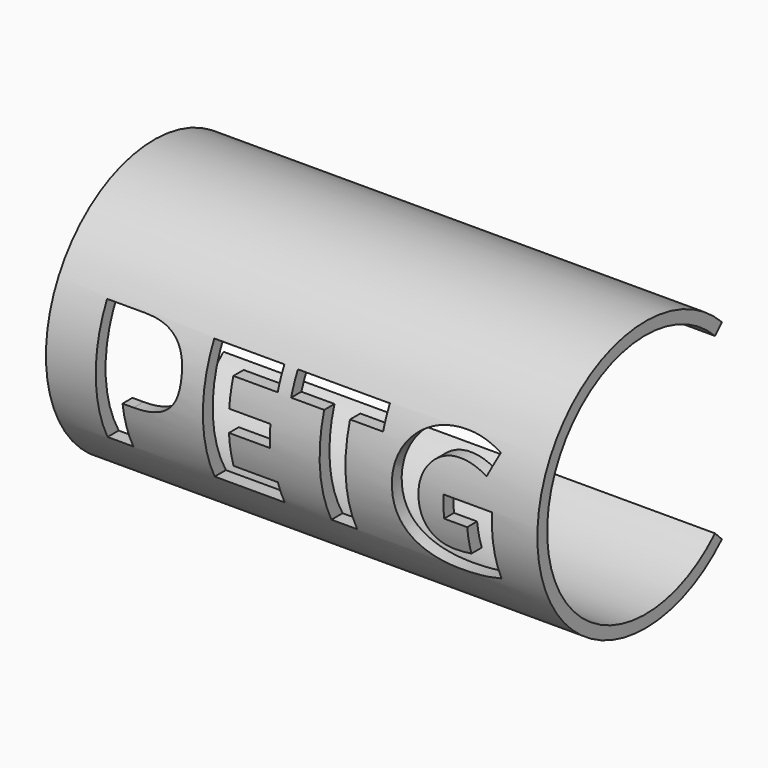
from build123d import *

# Parameters (mm, degrees)
F1_DEPTH     = 50.8
F3_TEXT_SIZE = 17.6388888889
F4_DEPTH     = 35.2792817332


# Not quite as in the source:
# - Text() gives the source's letters only with a copy of the font that has no kerning and outlines rounded to 1/6400 em; it was checked with that copy


with BuildPart() as f1:
    # F0 (on Right) → F1 (new body)
    with BuildSketch(Plane.YZ):
        with BuildLine():
            ThreePointArc((8.9802561211, -8.9802561211), (-12.7, 0), (8.9802561211, 8.9802561211))
            Line((8.9802561211, 8.9802561211), (9.8782817332, 9.8782817332))
            ThreePointArc((9.8782817332, 9.8782817332), (-13.97, 0), (9.8782817332, -9.8782817332))
            Line((9.8782817332, -9.8782817332), (8.9802561211, -8.9802561211))
        make_face()
    extrude(amount=F1_DEPTH)

    # F3 (on offset) → F4 (cut, through all)
    with BuildSketch(Plane.XZ.offset(25.4)):
        with Locations((3.5636067708, -6.35)):
            Text('PETG', F3_TEXT_SIZE, font='Open Sans', font_style=FontStyle.BOLD, text_align=(TextAlign.LEFT, TextAlign.BOTTOM))
        with BuildLine():
            Line((7.8189887153, 4.0541883681), (7.8189887153, 0.3169487847))
            Line((7.8189887153, 0.3169487847), (8.6981770833, 0.3169487847))
            add(Edge.make_bspline(
                [(8.6981770833, 0.3169487847), (9.9273871528, 0.3169487847), (10.5392361111, 0.8033962674)],
                knots=[0, 0, 0, 1, 1, 1], degree=2))
            add(Edge.make_bspline(
                [(10.5392361111, 0.8033962674), (11.1510850694, 1.28984375), (11.1510850694, 2.2186414931)],
                knots=[0, 0, 0, 1, 1, 1], degree=2))
            add(Edge.make_bspline(
                [(11.1510850694, 2.2186414931), (11.1510850694, 3.1584635417), (10.6384548611, 3.6063259549)],
                knots=[0, 0, 0, 1, 1, 1], degree=2))
            add(Edge.make_bspline(
                [(10.6384548611, 3.6063259549), (10.1258246528, 4.0541883681), (9.0316623264, 4.0541883681)],
                knots=[0, 0, 0, 1, 1, 1], degree=2))
            Line((9.0316623264, 4.0541883681), (7.8189887153, 4.0541883681))
        make_face()
    extrude(amount=-F4_DEPTH, mode=Mode.SUBTRACT)


solid = f1.part
